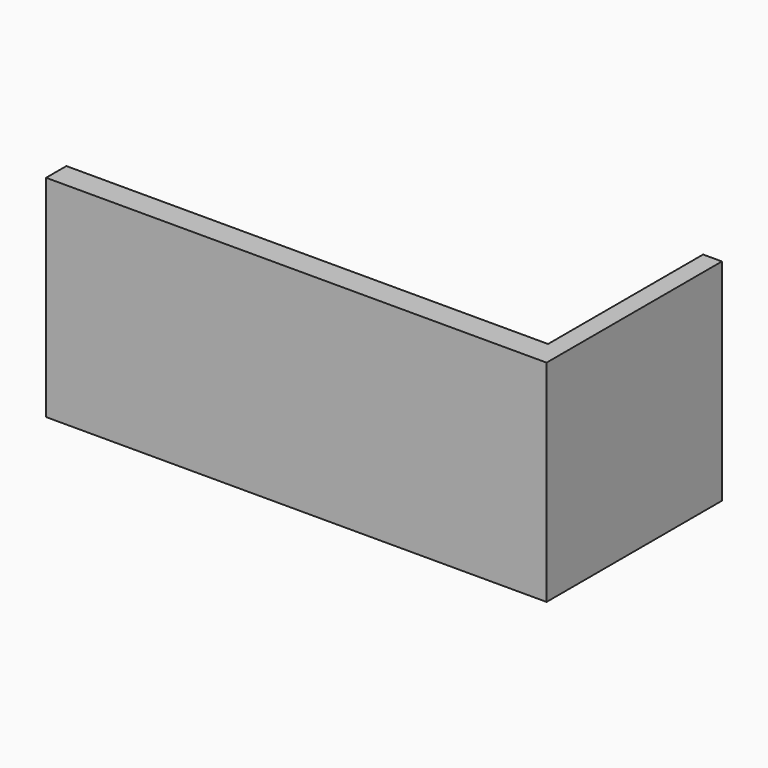
from build123d import *

# Parameters (mm, degrees)
F2_DEPTH = 76.2
F3_DEPTH = 76.2


# Not quite as in the source:
# - the program builds the solid bodies; features that only make, move or delete a surface that nothing else refers to are left out


with BuildPart() as f2:
    # F0 (on Top) → F2 (new body)
    with BuildSketch(Plane.XY):
        Polygon((88.587783277, 43.1846939027), (81.7847177386, 43.1846939027), (81.7847177386, -26.9164871424), (-92.4329981208, -26.9164871424), (-92.4329981208, -36.0858403146), (88.587783277, -36.0858403146), align=None)
    extrude(amount=F2_DEPTH)

    # F0 (on Top) → F3 (join)
    with BuildSketch(Plane.XY):
        Polygon((88.587783277, 43.1846939027), (81.7847177386, 43.1846939027), (81.7847177386, -26.9164871424), (-92.4329981208, -26.9164871424), (-92.4329981208, -36.0858403146), (88.587783277, -36.0858403146), align=None)
    extrude(amount=F3_DEPTH)


solid = f2.part
